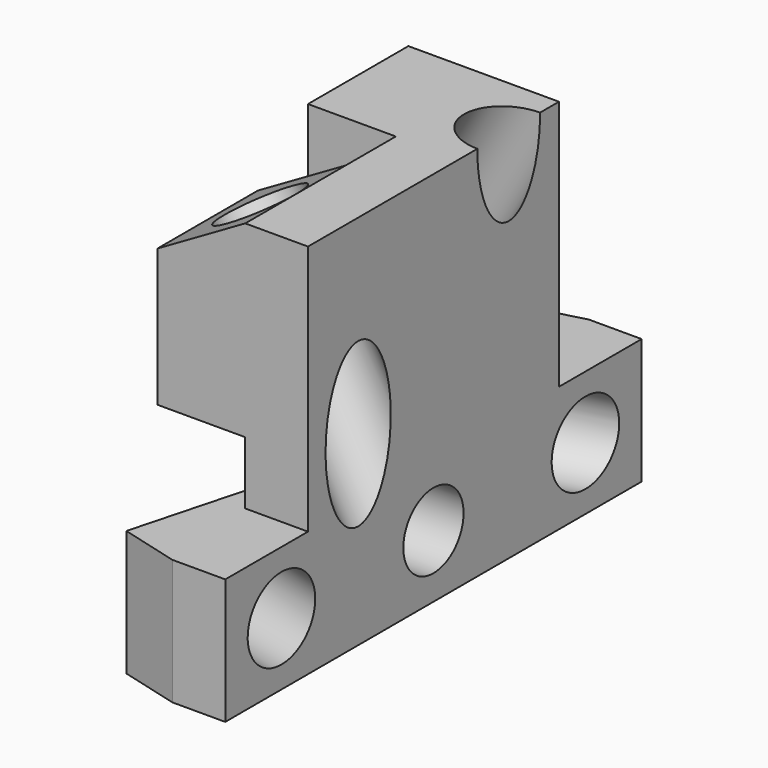
from build123d import *

# Parameters (mm, degrees)
F0_W          = 10
F0_H          = 5
F1_DEPTH      = 5
F1_DEPTH_BACK = 5
F2_R          = 1.75
F3_DEPTH      = 5
F5_DEPTH      = 10
F6_W          = 5
F6_H          = 10
F7_DEPTH      = 10
F8_R          = 3
F9_DEPTH      = 5
F10_R         = 3.25
F11_DEPTH     = 8.3257839131
F12_W         = 5
F12_H         = 25
F13_DEPTH     = 20
F15_DEPTH     = 10
F17_DEPTH     = 10
F18_W         = 7
F18_H         = 10
F19_DEPTH     = 5
F20_DEPTH     = 25
F21_R         = 3.25
F22_DEPTH     = 21.2593302492
F23_W         = 7
F23_H         = 10
F24_DEPTH     = 5
F25_R         = 3.125
F26_DEPTH     = 15.4913810568
F27_DEPTH     = 5.9595481157
F28_DEPTH     = 60.001
F29_DEPTH     = 30


# Not quite as in the source:
# - a pattern or mirror of a feature is missing from the dataset's text; its kind, count and spacing are read off the source's solid


with BuildPart() as f1:
    # F0 (on Front) → F1 (new body, two sides)
    with BuildSketch(Plane.XZ) as f1_sk:
        Rectangle(F0_W, F0_H)
    extrude(amount=F1_DEPTH)
    extrude(f1_sk.sketch, amount=-F1_DEPTH_BACK)

    # F2 (on face) → F3 (cut, through all)
    with BuildSketch(Plane.XY.offset(2.5)):
        Circle(F2_R)
    extrude(amount=-F3_DEPTH, mode=Mode.SUBTRACT)

    # F4 (on face) → F5 (join, through all)
    with BuildSketch(Plane.XZ.offset(5)):
        Polygon((-5, 2.5), (-10, 2.5), (-5, -2.5), align=None)
        Polygon((-10, 57.5), (-10, 2.5), (-5, 2.5), (-5, 27.5), (-5, 29.5), (-5, 55.5), (-5, 57.5), align=None)
        Polygon((-5, 29.5), (-5, 27.5), (23, 27.5), (23, 57.5), (-5, 57.5), (-5, 55.5), (21, 55.5), (21, 29.5), align=None)
    extrude(amount=-F5_DEPTH)

    # F6 (on face) → F7 (join)
    with BuildSketch(Plane.XY.offset(57.5)):
        with Locations((20.5, 0)):
            Rectangle(F6_W, F6_H)
        Polygon((18.7827778329, -20.7388873943), (23, -5), (18, -5), (14.1177143235, -19.4888873943), align=None)
        Polygon((18, 5), (23, 5), (18.7827778329, 20.7388873943), (14.1177143235, 19.4888873943), align=None)
        Polygon((23, -20.7388873943), (23, -5), (18.7827778329, -20.7388873943), align=None)
        Polygon((18.7827778329, 20.7388873943), (23, 5), (23, 20.7388873943), align=None)
    extrude(amount=F7_DEPTH)

    # F8 (on face) → F9 (cut, through all)
    with BuildSketch(Plane.YZ.offset(23)):
        with Locations((0, 62.5)):
            Circle(F8_R)
    extrude(amount=-F9_DEPTH, mode=Mode.SUBTRACT)

    # F10 (on face) → F11 (cut, through all)
    with BuildSketch(Plane(origin=(18.0442286341, -4.8349364905, 0), x_dir=(-0.2588190451, -0.9659258263, 0), z_dir=(-0.9659258263, 0.2588190451, 0))):
        with Locations((8.6708863196, 62.5)):
            Circle(F10_R)
    f11 = extrude(amount=-F11_DEPTH, mode=Mode.SUBTRACT)

    # F11_copies: F11 across plane
    add(f11.mirror(Plane.ZX.offset(-3e-06)), mode=Mode.SUBTRACT)

    # F12 (on face) → F13 (join)
    with BuildSketch(Plane.XY.offset(67.5)):
        with Locations((20.5, 0)):
            Rectangle(F12_W, F12_H)
    extrude(amount=F13_DEPTH)

    # F14 (on face) → F15 (join)
    with BuildSketch(Plane(origin=(0, 12.5, 0), x_dir=(-1, 0, 0), z_dir=(0, 1, 0))):
        Polygon((-18, 82.5), (-18, 72.5), (-0.6794919243, 82.5), align=None)
    extrude(amount=-F15_DEPTH)

    # F16 (on face) → F17 (join)
    with BuildSketch(Plane.XZ.offset(12.5)):
        Polygon((18, 77.5), (18, 87.5), (0.6794919243, 77.5), align=None)
    extrude(amount=-F17_DEPTH)

    # F18 (on face) → F19 (join)
    with BuildSketch(Plane(origin=(0, 0, 77.5), x_dir=(1, 0, 0), z_dir=(0, 0, -1))):
        with Locations((14.5, 7.5)):
            Rectangle(F18_W, F18_H)
    extrude(amount=F19_DEPTH)

    # F20 (cut): a face of the model
    f20_faces = [f1.faces().sort_by_distance(p)[0] for p in [
        (5.8397459622, -7.5, 77.5),
    ]]
    extrude(f20_faces, amount=-F20_DEPTH, mode=Mode.SUBTRACT)

    # F21 (on face) → F22 (cut, through all)
    with BuildSketch(Plane(origin=(-33.3886114156, 0, 57.8307713659), x_dir=(0.8660254038, 0, 0.5), z_dir=(-0.5, 0, 0.8660254038))):
        with Locations((56.0884572681, -7.5)):
            Circle(F21_R)
    extrude(amount=-F22_DEPTH, mode=Mode.SUBTRACT)

    # F23 (on face) → F24 (join)
    with BuildSketch(Plane.XY.offset(82.5)):
        with Locations((14.5, 7.5)):
            Rectangle(F23_W, F23_H)
    extrude(amount=F24_DEPTH)

    # F25 (on face) → F26 (cut, through all)
    with BuildSketch(Plane(origin=(35.8934208872, 0, 62.1692286341), x_dir=(0.8660254038, 0, -0.5), z_dir=(-0.5, 0, -0.8660254038))):
        with Locations((-23.7865427319, -7.5)):
            Circle(F25_R)
    extrude(amount=-F26_DEPTH, mode=Mode.SUBTRACT)

    # F27 (cut, through all): a face of the model
    f27_faces = [f1.faces().sort_by_distance(p)[0] for p in [
        (5.8397459622, 7.5, 82.5),
    ]]
    extrude(f27_faces, amount=-F27_DEPTH, mode=Mode.SUBTRACT)

    # F28 (cut, through all): a face of the model
    f28_faces = [f1.faces().sort_by_distance(p)[0] for p in [
        (4, 0, 57.5),
    ]]
    extrude(f28_faces, amount=-F28_DEPTH, mode=Mode.SUBTRACT)

    # F29 (cut, through all): a face of the model
    f29_faces = [f1.faces().sort_by_distance(p)[0] for p in [
        (20.5, 0, 27.5),
    ]]
    extrude(f29_faces, amount=-F29_DEPTH, mode=Mode.SUBTRACT)


solid = f1.part
